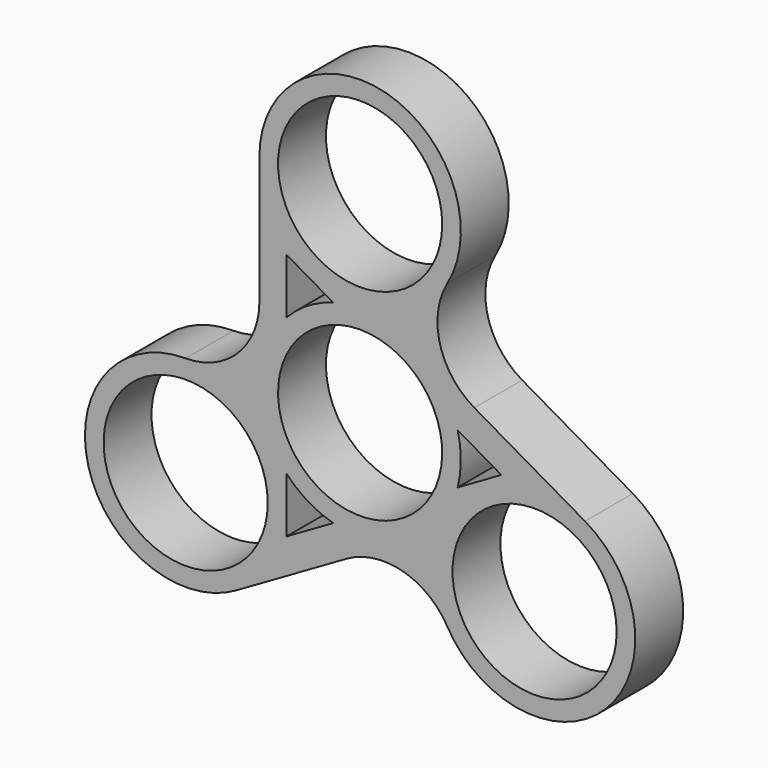
from build123d import *

# Parameters (mm, degrees)
F1_R     = 9.6120137511
F2_DEPTH = 7.0104


# Not quite as in the source:
# - a variable given as a bare number and used for a length is read in inches; the dataset says mm whatever the document's units were


with BuildPart() as f2:
    # F1 (on Front) → F2 (new body)
    with BuildSketch(Plane.XZ):
        with BuildLine():
            ThreePointArc((-1.5804976935, -14.5344976935), (4.97266358, -13.6717576448), (10.2164976935, -17.6954930806))
            ThreePointArc((10.2164976935, -17.6954930806), (28.7747308229, -20.1387308229), (26.3314930806, -1.5804976935))
            Line((26.3314930806, -1.5804976935), (13.3774930806, 5.8984976935))
            ThreePointArc((13.3774930806, 5.8984976935), (9.3537576448, 11.1423318071), (10.2164976935, 17.6954930806))
            ThreePointArc((10.2164976935, 17.6954930806), (3.0532870812, 34.9890132912), (-11.7969953871, 23.5939907742))
            Line((-11.7969953871, 23.5939907742), (-11.7969953871, 8.636))
            ThreePointArc((-11.7969953871, 8.636), (-14.3264212248, 2.5294258377), (-20.4329953871, 0))
            ThreePointArc((-20.4329953871, 0), (-31.8280179041, -14.8502824682), (-14.5344976935, -22.0134930806))
            Line((-14.5344976935, -22.0134930806), (-1.5804976935, -14.5344976935))
        make_face()
        with Locations((-20.4329953871, -11.7969953871)):
            Circle(F1_R, mode=Mode.SUBTRACT)
        with BuildLine():
            Line((-8.636, -14.5344976935), (-8.636, -8.0367035632))
            ThreePointArc((-8.636, -8.0367035632), (-6.1247501657, -10.0824865768), (-3.1517710218, -11.3681766167))
            Line((-3.1517710218, -11.3681766167), (-8.636, -14.5344976935))
        make_face(mode=Mode.SUBTRACT)
        with Locations((20.4329953871, -11.7969953871)):
            Circle(F1_R, mode=Mode.SUBTRACT)
        with BuildLine():
            ThreePointArc((-0.1089384298, 9.6113964006), (6.7580948005, 6.8351271399), (9.6120137511, 0))
            ThreePointArc((9.6120137511, 0), (9.2984411415, -2.4351182085), (8.3781826637, -4.7113547526))
            ThreePointArc((8.3781826637, -4.7113547526), (-0.2773430479, -9.6080117186), (-8.636, -4.2202265758))
            ThreePointArc((-8.636, -4.2202265758), (-8.1821107042, 5.0441919844), (-0.1089384298, 9.6113964006))
        make_face(mode=Mode.SUBTRACT)
        with BuildLine():
            Line((11.4210152557, 2.9545745365), (16.5384884677, 0))
            Line((16.5384884677, 0), (11.4210152557, -2.9545745365))
            ThreePointArc((11.4210152557, -2.9545745365), (11.7969953871, 0), (11.4210152557, 2.9545745365))
        make_face(mode=Mode.SUBTRACT)
        with BuildLine():
            Line((-8.636, 8.0367035632), (-8.636, 14.5344976935))
            Line((-8.636, 14.5344976935), (-3.1517710218, 11.3681766167))
            ThreePointArc((-3.1517710218, 11.3681766167), (-6.1247501657, 10.0824865768), (-8.636, 8.0367035632))
        make_face(mode=Mode.SUBTRACT)
        with Locations((0, 23.5939907742)):
            Circle(F1_R, mode=Mode.SUBTRACT)
    extrude(amount=F2_DEPTH)


solid = f2.part
